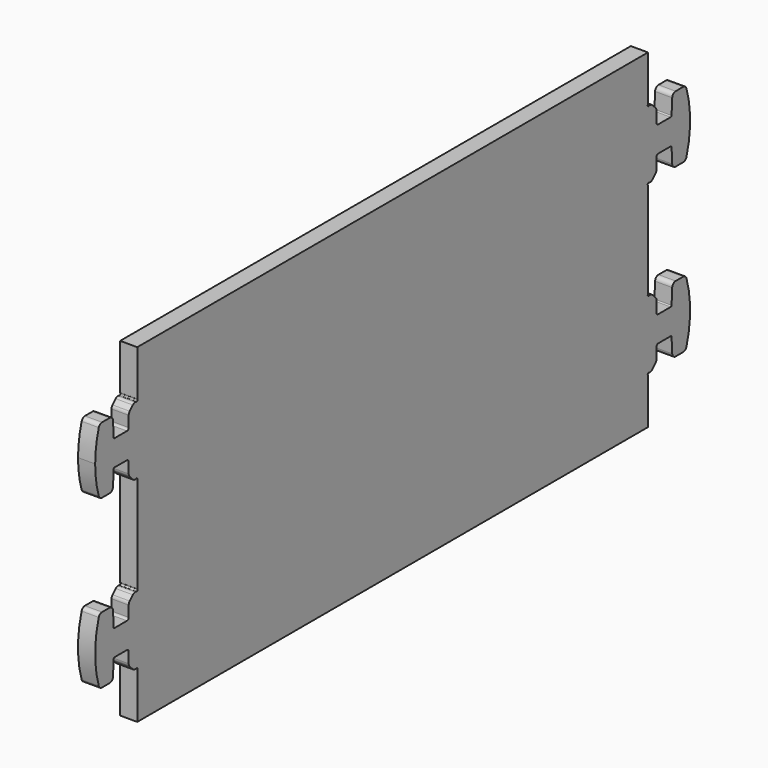
from build123d import *

# Parameters (mm, degrees)
F1_DEPTH = 12.7


# Not quite as in the source:
# - ends of sketch curves that miss each other by under 0.0002 mm in the source are joined


with BuildPart() as f1:
    # F0 (on Right) → F1 (new body)
    with BuildSketch(Plane.YZ):
        with BuildLine():
            Line((236.5375, -109.1388978), (236.5375, -75.4041672))
            ThreePointArc((236.5375, -75.4041672), (236.5078654625, -75.1891279146), (236.4211711171, -74.9901198984))
            ThreePointArc((236.4211711171, -74.9901198984), (236.3106086135, -74.4826598929), (236.5374977924, -74.0154707924))
            ThreePointArc((236.5374977924, -74.0154707924), (237.0047819511, -73.7885702728), (237.5123174318, -73.8992322198))
            ThreePointArc((237.5123174318, -73.8992322198), (237.7110840704, -73.9858367525), (237.925864, -74.0154476))
            Line((237.925864, -74.0154476), (238.3973642, -74.015473))
            ThreePointArc((238.3973642, -74.015473), (239.6123840978, -73.7737651157), (240.6424282303, -73.0855116303))
            Line((240.6424282303, -73.0855116303), (243.5450552, -70.1828924))
            ThreePointArc((243.5450552, -70.1828924), (244.2333175157, -69.1528570978), (244.475, -67.9378372))
            Line((244.475, -67.9378372), (244.475, -59.9263978))
            ThreePointArc((244.475, -59.9263978), (244.9399679849, -58.8038657849), (246.0625, -58.3388978))
            Line((246.0625, -58.3388978), (257.6125404, -58.3388978))
            ThreePointArc((257.6125404, -58.3388978), (258.1588619483, -58.5568250596), (258.4051939334, -59.0909412245))
            Line((258.4051939334, -59.0909412245), (259.0010568, -70.4120258))
            ThreePointArc((259.0010568, -70.4120258), (259.986395292, -72.5484566791), (262.1716626, -73.4201478))
            Line((262.1716626, -73.4201478), (269.1608282, -73.4201478))
            ThreePointArc((269.1608282, -73.4201478), (271.0444892731, -72.8010128124), (272.1935106769, -71.1850743899))
            ThreePointArc((272.1935106769, -71.1850743899), (275.5807798, -48.8138978), (272.193515932, -26.4427195814))
            ThreePointArc((272.193515932, -26.4427195814), (271.0444892731, -24.8267827876), (269.1608282, -24.2076478))
            Line((269.1608282, -24.2076478), (262.1716626, -24.2076478))
            ThreePointArc((262.1716626, -24.2076478), (259.986395292, -25.0793389209), (259.0010512024, -27.2157695054))
            Line((259.0010512024, -27.2157695054), (258.4051982, -38.5368546))
            ThreePointArc((258.4051982, -38.5368546), (258.1588619483, -39.0709705404), (257.6125404, -39.2888978))
            Line((257.6125404, -39.2888978), (246.0625, -39.2888978))
            ThreePointArc((246.0625, -39.2888978), (244.9399679849, -38.8239298151), (244.475, -37.7013978))
            Line((244.475, -37.7013978), (244.475, -29.6899584))
            ThreePointArc((244.475, -29.6899584), (244.2333175157, -28.4749385022), (243.5450640303, -27.4448943697))
            Line((243.5450640303, -27.4448943697), (240.6424448, -24.5422674))
            ThreePointArc((240.6424448, -24.5422674), (239.6123923944, -23.8540085209), (238.3973642, -23.6123226))
            Line((238.3973642, -23.6123226), (237.9262196, -23.6123226))
            ThreePointArc((237.9262196, -23.6123226), (237.7111803146, -23.6419825375), (237.5121722984, -23.7286768829))
            ThreePointArc((237.5121722984, -23.7286768829), (236.5375007816, -23.6123277967), (236.4211594841, -22.6376686047))
            ThreePointArc((236.4211594841, -22.6376686047), (236.5078654625, -22.4386676854), (236.5375, -22.2236284))
            Line((236.5375, -22.2236284), (236.5375, 48.4208328))
            ThreePointArc((236.5375, 48.4208328), (236.5078654625, 48.6358720854), (236.4211711171, 48.8348801016))
            ThreePointArc((236.4211711171, 48.8348801016), (236.5375007816, 49.8095321967), (237.5121612128, 49.9258631126))
            ThreePointArc((237.5121612128, 49.9258631126), (237.7111739468, 49.8391633266), (237.9262196, 49.809527))
            Line((237.9262196, 49.809527), (238.3973642, 49.809527))
            ThreePointArc((238.3973642, 49.809527), (239.6123923944, 50.0512129209), (240.6424409302, 50.7394756697))
            Line((240.6424409302, 50.7394756697), (243.5450552, 53.6421076))
            ThreePointArc((243.5450552, 53.6421076), (244.2333175157, 54.6721429022), (244.475, 55.8871628))
            Line((244.475, 55.8871628), (244.475, 63.8986022))
            ThreePointArc((244.475, 63.8986022), (244.9399679849, 65.0211342151), (246.0625, 65.4861022))
            Line((246.0625, 65.4861022), (257.6125404, 65.4861022))
            ThreePointArc((257.6125404, 65.4861022), (258.1588619483, 65.2681749404), (258.4051939334, 64.7340587755))
            Line((258.4051939334, 64.7340587755), (259.0010568, 53.4129742))
            ThreePointArc((259.0010568, 53.4129742), (259.986395292, 51.2765433209), (262.1716626, 50.4048522))
            Line((262.1716626, 50.4048522), (269.1608282, 50.4048522))
            ThreePointArc((269.1608282, 50.4048522), (271.0444892731, 51.0239871876), (272.1935106769, 52.6399256101))
            ThreePointArc((272.1935106769, 52.6399256101), (275.5807798, 75.0111022), (272.193515932, 97.3822804186))
            ThreePointArc((272.193515932, 97.3822804186), (271.0444892731, 98.9982172124), (269.1608282, 99.6173522))
            Line((269.1608282, 99.6173522), (262.1716626, 99.6173522))
            ThreePointArc((262.1716626, 99.6173522), (259.986395292, 98.7456610791), (259.0010512024, 96.6092304946))
            Line((259.0010512024, 96.6092304946), (258.4051982, 85.2881454))
            ThreePointArc((258.4051982, 85.2881454), (258.1588619483, 84.7540294596), (257.6125404, 84.5361022))
            Line((257.6125404, 84.5361022), (246.0625, 84.5361022))
            ThreePointArc((246.0625, 84.5361022), (244.9399679849, 85.0010701849), (244.475, 86.1236022))
            Line((244.475, 86.1236022), (244.475, 94.1350416))
            ThreePointArc((244.475, 94.1350416), (244.2333175157, 95.3500614978), (243.5450640303, 96.3801056303))
            Line((243.5450640303, 96.3801056303), (240.6424448, 99.2827326))
            ThreePointArc((240.6424448, 99.2827326), (239.6123840978, 99.9709695157), (238.3973642, 100.212652))
            Line((238.3973642, 100.212652), (237.925864, 100.2126774))
            ThreePointArc((237.925864, 100.2126774), (237.7110777005, 100.183064762), (237.5123175778, 100.0964363809))
            ThreePointArc((237.5123175778, 100.0964363809), (237.0047819511, 99.9857746728), (236.5374977924, 100.2126751924))
            ThreePointArc((236.5374977924, 100.2126751924), (236.3106086135, 100.6798642929), (236.4211594841, 101.1873313953))
            ThreePointArc((236.4211594841, 101.1873313953), (236.5078654625, 101.3863323146), (236.5375, 101.6013716))
            Line((236.5375, 101.6013716), (236.5375, 135.3361022))
            Line((236.5375, 135.3361022), (-236.5375, 135.3361022))
            Line((-236.5375, 135.3361022), (-236.5375, 101.6013716))
            ThreePointArc((-236.5375, 101.6013716), (-236.5078654625, 101.3863323146), (-236.4211711171, 101.1873242984))
            ThreePointArc((-236.4211711171, 101.1873242984), (-236.3106086135, 100.6798642929), (-236.5374977924, 100.2126751924))
            ThreePointArc((-236.5374977924, 100.2126751924), (-237.0047819511, 99.9857746728), (-237.5123174318, 100.0964366198))
            ThreePointArc((-237.5123174318, 100.0964366198), (-237.7110840704, 100.1830411525), (-237.925864, 100.212652))
            Line((-237.925864, 100.212652), (-238.3973642, 100.2126774))
            ThreePointArc((-238.3973642, 100.2126774), (-239.6123923944, 99.9709914791), (-240.6424409302, 99.2827287303))
            Line((-240.6424409302, 99.2827287303), (-243.5450552, 96.3800968))
            ThreePointArc((-243.5450552, 96.3800968), (-244.2333175157, 95.3500614978), (-244.475, 94.1350416))
            Line((-244.475, 94.1350416), (-244.475, 86.1236022))
            ThreePointArc((-244.475, 86.1236022), (-244.9399679849, 85.0010701849), (-246.0625, 84.5361022))
            Line((-246.0625, 84.5361022), (-257.6125404, 84.5361022))
            ThreePointArc((-257.6125404, 84.5361022), (-258.1588619483, 84.7540294596), (-258.4051939334, 85.2881456245))
            Line((-258.4051939334, 85.2881456245), (-259.0010568, 96.6092302))
            ThreePointArc((-259.0010568, 96.6092302), (-259.986395292, 98.7456610791), (-262.1716626, 99.6173522))
            Line((-262.1716626, 99.6173522), (-269.1608282, 99.6173522))
            ThreePointArc((-269.1608282, 99.6173522), (-271.0444892731, 98.9982172124), (-272.1935106769, 97.3822787899))
            ThreePointArc((-272.1935106769, 97.3822787899), (-274.6753600499, 86.3180167058), (-275.5304647976, 75.0111022805))
            ThreePointArc((-275.5304647976, 75.0111022805), (-274.7326706384, 63.6956391914), (-272.1935194926, 52.639922854))
            ThreePointArc((-272.1935194926, 52.639922854), (-271.0444892731, 51.0239871876), (-269.1608282, 50.4048522))
            Line((-269.1608282, 50.4048522), (-262.1716626, 50.4048522))
            ThreePointArc((-262.1716626, 50.4048522), (-259.986395292, 51.2765433209), (-259.0010512024, 53.4129739054))
            Line((-259.0010512024, 53.4129739054), (-258.4051982, 64.734059))
            ThreePointArc((-258.4051982, 64.734059), (-258.1588619483, 65.2681749404), (-257.6125404, 65.4861022))
            Line((-257.6125404, 65.4861022), (-246.0625, 65.4861022))
            ThreePointArc((-246.0625, 65.4861022), (-244.9399679849, 65.0211342151), (-244.475, 63.8986022))
            Line((-244.475, 63.8986022), (-244.475, 55.8871628))
            ThreePointArc((-244.475, 55.8871628), (-244.2333175157, 54.6721429022), (-243.5450640303, 53.6420987697))
            Line((-243.5450640303, 53.6420987697), (-240.6424448, 50.7394718))
            ThreePointArc((-240.6424448, 50.7394718), (-239.6123923944, 50.0512129209), (-238.3973642, 49.809527))
            Line((-238.3973642, 49.809527), (-237.9262196, 49.809527))
            ThreePointArc((-237.9262196, 49.809527), (-237.7111803146, 49.8391869375), (-237.5121722984, 49.9258812829))
            ThreePointArc((-237.5121722984, 49.9258812829), (-236.5375007816, 49.8095321967), (-236.4211594841, 48.8348730047))
            ThreePointArc((-236.4211594841, 48.8348730047), (-236.5078654625, 48.6358720854), (-236.5375, 48.4208328))
            Line((-236.5375, 48.4208328), (-236.5375, -22.2236284))
            ThreePointArc((-236.5375, -22.2236284), (-236.5078654625, -22.4386676854), (-236.4211711171, -22.6376757016))
            ThreePointArc((-236.4211711171, -22.6376757016), (-236.5375007816, -23.6123277967), (-237.5121612128, -23.7286587126))
            ThreePointArc((-237.5121612128, -23.7286587126), (-237.7111739468, -23.6419589266), (-237.9262196, -23.6123226))
            Line((-237.9262196, -23.6123226), (-238.3973642, -23.6123226))
            ThreePointArc((-238.3973642, -23.6123226), (-239.6123923944, -23.8540085209), (-240.6424409302, -24.5422712697))
            Line((-240.6424409302, -24.5422712697), (-243.5450552, -27.4449032))
            ThreePointArc((-243.5450552, -27.4449032), (-244.2333175157, -28.4749385022), (-244.475, -29.6899584))
            Line((-244.475, -29.6899584), (-244.475, -37.7013978))
            ThreePointArc((-244.475, -37.7013978), (-244.9399679849, -38.8239298151), (-246.0625, -39.2888978))
            Line((-246.0625, -39.2888978), (-257.6125404, -39.2888978))
            ThreePointArc((-257.6125404, -39.2888978), (-258.1588619483, -39.0709705404), (-258.4051939334, -38.5368543755))
            Line((-258.4051939334, -38.5368543755), (-259.0010568, -27.2157698))
            ThreePointArc((-259.0010568, -27.2157698), (-259.986395292, -25.0793389209), (-262.1716626, -24.2076478))
            Line((-262.1716626, -24.2076478), (-269.1608282, -24.2076478))
            ThreePointArc((-269.1608282, -24.2076478), (-271.0444892731, -24.8267827876), (-272.1935106769, -26.4427212101))
            ThreePointArc((-272.1935106769, -26.4427212101), (-275.5807798, -48.8138978), (-272.193515932, -71.1850760186))
            ThreePointArc((-272.193515932, -71.1850760186), (-271.0444892731, -72.8010128124), (-269.1608282, -73.4201478))
            Line((-269.1608282, -73.4201478), (-262.1716626, -73.4201478))
            ThreePointArc((-262.1716626, -73.4201478), (-259.986395292, -72.5484566791), (-259.0010512024, -70.4120260946))
            Line((-259.0010512024, -70.4120260946), (-258.4051982, -59.090941))
            ThreePointArc((-258.4051982, -59.090941), (-258.1588619483, -58.5568250596), (-257.6125404, -58.3388978))
            Line((-257.6125404, -58.3388978), (-246.0625, -58.3388978))
            ThreePointArc((-246.0625, -58.3388978), (-244.9399679849, -58.8038657849), (-244.475, -59.9263978))
            Line((-244.475, -59.9263978), (-244.475, -67.9378372))
            ThreePointArc((-244.475, -67.9378372), (-244.2333175157, -69.1528570978), (-243.5450640303, -70.1829012303))
            Line((-243.5450640303, -70.1829012303), (-240.6424448, -73.0855282))
            ThreePointArc((-240.6424448, -73.0855282), (-239.6123923944, -73.7737870791), (-238.3973642, -74.015473))
            Line((-238.3973642, -74.015473), (-237.925864, -74.015473))
            ThreePointArc((-237.925864, -74.015473), (-237.7110777005, -73.985860362), (-237.5123175778, -73.8992319809))
            ThreePointArc((-237.5123175778, -73.8992319809), (-237.0047819511, -73.7885702728), (-236.5374977924, -74.0154707924))
            ThreePointArc((-236.5374977924, -74.0154707924), (-236.3106086135, -74.4826598929), (-236.4211594841, -74.9901269953))
            ThreePointArc((-236.4211594841, -74.9901269953), (-236.5078654625, -75.1891279146), (-236.5375, -75.4041672))
            Line((-236.5375, -75.4041672), (-236.5375, -109.1388978))
            Line((-236.5375, -109.1388978), (236.5375, -109.1388978))
        make_face()
    extrude(amount=F1_DEPTH)


solid = f1.part
